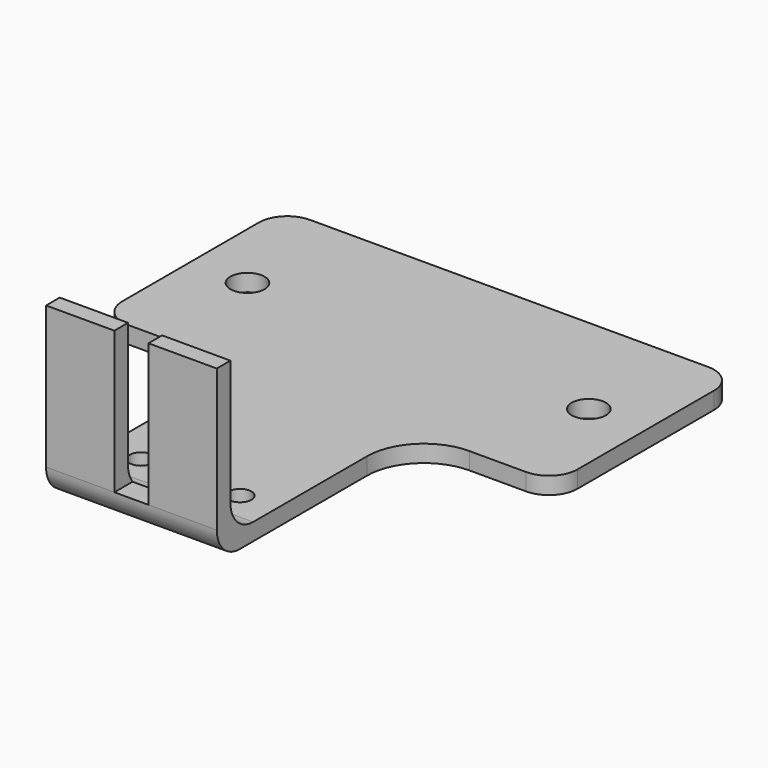
from build123d import *

# Parameters (mm, degrees)
F1_DEPTH     = 3
F2_D         = 4
F3_D         = 6
F5_W         = 30
F5_H         = 3
F6_DEPTH     = 3
F7_T4_DEPTH  = 30
F7_T10_DEPTH = 30
F7_T16_DEPTH = 30
F7_T23_DEPTH = 30
F7_T29_DEPTH = 30
F7_T32_DEPTH = 55


# Not quite as in the source:
# - a fillet or chamfer that OpenCascade refuses, or shapes differently, is made with other operations: its cross-section is extruded or revolved along the edge and cut away or added


with BuildPart() as f1:
    # F0 (on Top) → F1 (new body)
    with BuildSketch(Plane.XY):
        with BuildLine():
            Line((40.0588317961, -2.3308048306), (-29.9411682039, -2.3308048306))
            ThreePointArc((-29.9411682039, -2.3308048306), (-33.4767021099, -3.7952709247), (-34.9411682039, -7.3308048306))
            Line((-34.9411682039, -7.3308048306), (-34.9411682039, -37.3308048306))
            ThreePointArc((-34.9411682039, -37.3308048306), (-33.4767021099, -40.8663387365), (-29.9411682039, -42.3308048306))
            Line((-29.9411682039, -42.3308048306), (-19.9411682039, -42.3308048306))
            ThreePointArc((-19.9411682039, -42.3308048306), (-12.8701003921, -45.2597370187), (-9.9411682039, -52.3308048306))
            Line((-9.9411682039, -52.3308048306), (-9.9411682039, -82.3308048306))
            Line((-9.9411682039, -82.3308048306), (5.0588317961, -82.3308048306))
            Line((5.0588317961, -82.3308048306), (20.0588317961, -82.3308048306))
            Line((20.0588317961, -82.3308048306), (20.0588317961, -52.3308048306))
            ThreePointArc((20.0588317961, -52.3308048306), (22.9877639842, -45.2597370187), (30.0588317961, -42.3308048306))
            Line((30.0588317961, -42.3308048306), (40.0588317961, -42.3308048306))
            ThreePointArc((40.0588317961, -42.3308048306), (43.594365702, -40.8663387365), (45.0588317961, -37.3308048306))
            Line((45.0588317961, -37.3308048306), (45.0588317961, -7.3308048306))
            ThreePointArc((45.0588317961, -7.3308048306), (43.594365702, -3.7952709247), (40.0588317961, -2.3308048306))
        make_face()
    extrude(amount=F1_DEPTH)

    # F2 (through all)
    with Locations(Plane(origin=(0, 0, 0), x_dir=(1, 0, 0), z_dir=(0, 0, -1))):
        with Locations((-3.6411682039, 72.3308048306), (13.7588317961, 72.3308048306)):
            Hole(F2_D / 2)

    # F3 (through all)
    with Locations(Plane(origin=(0, 0, 0), x_dir=(1, 0, 0), z_dir=(0, 0, -1))):
        with Locations((-24.9411682039, 22.3308048306), (35.0588317961, 22.3308048306)):
            Hole(F3_D / 2)

    # F5 (on face) → F6 (join)
    with BuildSketch(Plane.XZ.offset(82.3308048306)):
        Polygon((-9.9411682039, 30), (-9.9411682039, 3), (20.0588317961, 3), (20.0588317961, 30), (8.0588317961, 30), (8.0588317961, 5), (2.0588317961, 5), (2.0588317961, 30), align=None)
        with Locations((5.0588317961, 1.5)):
            Rectangle(F5_W, F5_H)
    extrude(amount=F6_DEPTH)

    # F7: fillet of radius 5 on 2 edges, made by hand


with BuildPart() as f7_tool2:
    # F7_s3 → F7_t4 (new body)
    with BuildSketch(Plane.YZ.offset(20.0588317961)):
        with BuildLine():
            ThreePointArc((-77.3308048306, 3), (-80.8663387365, 4.4644660941), (-82.3308048306, 8))
            Line((-82.3308048306, 8), (-82.3308048306, 3))
            Line((-82.3308048306, 3), (-77.3308048306, 3))
        make_face()
    extrude(amount=-F7_T4_DEPTH)

    split(bisect_by=Plane.XY.offset(5), keep=Keep.BOTTOM)

    split(bisect_by=Plane.YZ.offset(8.0588317961), keep=Keep.TOP)


with BuildPart() as f1_1:
    add(f1.part)

    # F7_t1: union F7_tool2
    add(f7_tool2.part)


with BuildPart() as f7_tool8:
    # F7_s9 → F7_t10 (new body)
    with BuildSketch(Plane.YZ.offset(20.0588317961)):
        with BuildLine():
            ThreePointArc((-77.3308048306, 3), (-80.8663387365, 4.4644660941), (-82.3308048306, 8))
            Line((-82.3308048306, 8), (-82.3308048306, 3))
            Line((-82.3308048306, 3), (-77.3308048306, 3))
        make_face()
    extrude(amount=-F7_T10_DEPTH)

    split(bisect_by=Plane.XY.offset(5), keep=Keep.TOP)

    split(bisect_by=Plane.YZ.offset(8.0588317961), keep=Keep.TOP)


with BuildPart() as f1_2:
    add(f1_1.part)

    # F7_t7: union F7_tool8
    add(f7_tool8.part)


with BuildPart() as f7_tool14:
    # F7_s15 → F7_t16 (new body)
    with BuildSketch(Plane.YZ.offset(20.0588317961)):
        with BuildLine():
            ThreePointArc((-77.3308048306, 3), (-80.8663387365, 4.4644660941), (-82.3308048306, 8))
            Line((-82.3308048306, 8), (-82.3308048306, 3))
            Line((-82.3308048306, 3), (-77.3308048306, 3))
        make_face()
    extrude(amount=-F7_T16_DEPTH)

    split(bisect_by=Plane.YZ.offset(2.0588317961), keep=Keep.TOP)

    split(bisect_by=Plane.XY.offset(5), keep=Keep.BOTTOM)

    split(bisect_by=Plane.YZ.offset(8.0588317961), keep=Keep.BOTTOM)


with BuildPart() as f1_3:
    add(f1_2.part)

    # F7_t13: union F7_tool14
    add(f7_tool14.part)


with BuildPart() as f7_tool21:
    # F7_s22 → F7_t23 (new body)
    with BuildSketch(Plane.YZ.offset(20.0588317961)):
        with BuildLine():
            ThreePointArc((-77.3308048306, 3), (-80.8663387365, 4.4644660941), (-82.3308048306, 8))
            Line((-82.3308048306, 8), (-82.3308048306, 3))
            Line((-82.3308048306, 3), (-77.3308048306, 3))
        make_face()
    extrude(amount=-F7_T23_DEPTH)

    split(bisect_by=Plane.YZ.offset(2.0588317961), keep=Keep.BOTTOM)

    split(bisect_by=Plane.XY.offset(5), keep=Keep.BOTTOM)


with BuildPart() as f1_4:
    add(f1_3.part)

    # F7_t20: union F7_tool21
    add(f7_tool21.part)


with BuildPart() as f7_tool27:
    # F7_s28 → F7_t29 (new body)
    with BuildSketch(Plane.YZ.offset(20.0588317961)):
        with BuildLine():
            ThreePointArc((-77.3308048306, 3), (-80.8663387365, 4.4644660941), (-82.3308048306, 8))
            Line((-82.3308048306, 8), (-82.3308048306, 3))
            Line((-82.3308048306, 3), (-77.3308048306, 3))
        make_face()
    extrude(amount=-F7_T29_DEPTH)

    split(bisect_by=Plane.YZ.offset(2.0588317961), keep=Keep.BOTTOM)

    split(bisect_by=Plane.XY.offset(5), keep=Keep.TOP)


with BuildPart() as f1_5:
    add(f1_4.part)

    # F7_t26: union F7_tool27
    add(f7_tool27.part)

    # F7_s33 → F7_t32 (cut)
    with BuildSketch(Plane.YZ.offset(-22.4411682039)):
        with BuildLine():
            ThreePointArc((-85.3308048306, 5), (-83.8663387365, 1.4644660941), (-80.3308048306, 0))
            Line((-80.3308048306, 0), (-85.3308048306, 0))
            Line((-85.3308048306, 0), (-85.3308048306, 5))
        make_face()
    extrude(amount=F7_T32_DEPTH, mode=Mode.SUBTRACT)


solid = f1_5.part
